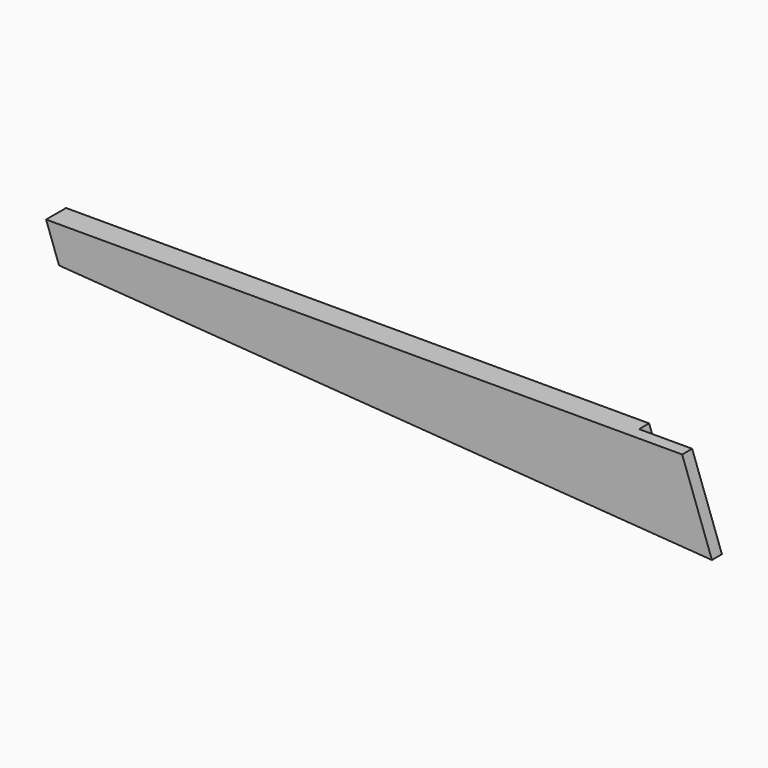
from build123d import *

# Parameters (mm, degrees)
F0_W     = 508
F0_H     = 63.5
F1_DEPTH = 19.05
F3_DEPTH = 50.8
F5_DEPTH = 50.8
F7_DEPTH = 38.1
F9_DEPTH = 38.1


with BuildPart() as f1:
    # F0 (on Front) → F1 (new body)
    with BuildSketch(Plane.XZ):
        with Locations((7.0352284261, 31.75)):
            Rectangle(F0_W, F0_H)
    extrude(amount=F1_DEPTH)

    # F2 (on face) → F3 (cut)
    with BuildSketch(Plane.XZ.offset(19.05)):
        Polygon((-224.2599035735, 0), (-246.9647715739, 63.5), (-246.9647715739, 0), align=None)
    extrude(amount=-F3_DEPTH, mode=Mode.SUBTRACT)

    # F4 (on face) → F5 (cut)
    with BuildSketch(Plane.XZ.offset(19.05)):
        Polygon((261.0352284261, 0), (-237.0874956021, 35.8756586385), (-224.2599035735, 0), align=None)
    extrude(amount=-F5_DEPTH, mode=Mode.SUBTRACT)

    # F6 (on face) → F7 (cut)
    with BuildSketch(Plane.XZ.offset(19.05)):
        Polygon((238.3303604257, 63.5), (261.0352284261, 0), (261.0352284261, 63.5), align=None)
    extrude(amount=-F7_DEPTH, mode=Mode.SUBTRACT)

    # F8 (on face) → F9 (cut)
    with BuildSketch(Plane(origin=(231.445604258, 0, 82.7549904558), x_dir=(0, 1, 0), z_dir=(0.941618337, 0, 0.3366822055))):
        Polygon((-9.525, 4.1548628118), (-9.525, -87.885916413), (0, -87.885916413), (0, 40.5242251848), align=None)
    extrude(amount=-F9_DEPTH, mode=Mode.SUBTRACT)


solid = f1.part
